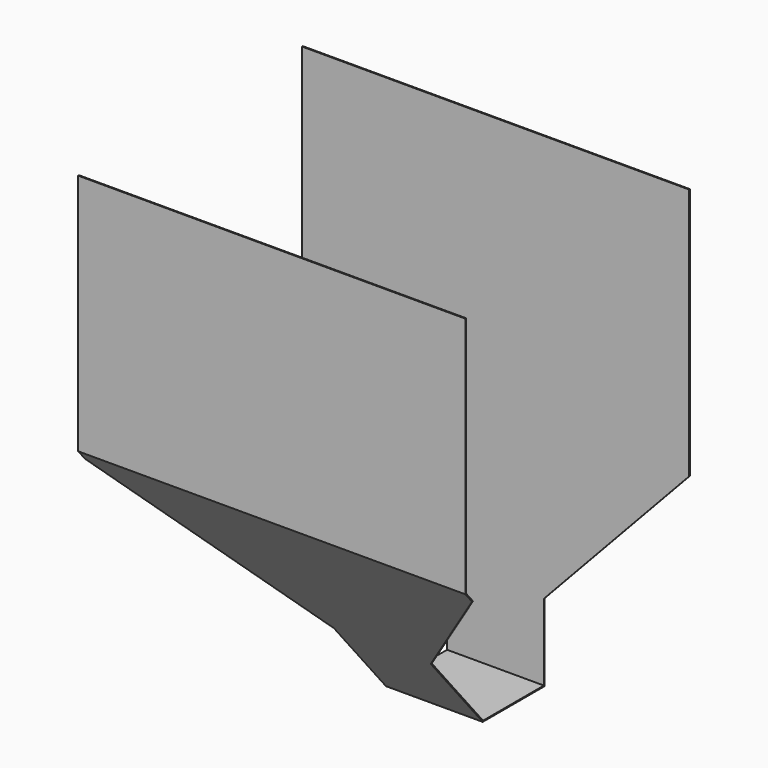
from build123d import *

# Parameters (mm, degrees)
F1_DEPTH = 400
F3_DEPTH = 290.001


# Not quite as in the source:
# - a feature names something its author has since deleted; it is built from what else it names


with BuildPart() as f1:
    # F0 (on Right) → F1 (new body)
    with BuildSketch(Plane.YZ):
        Polygon((-80, 0), (0, 0), (0, 501), (-1, 501), (-1, 1), (-79.5336923418, 1), (-289, 250.6322246791), (-289, 501), (-290, 501), (-290, 250.2682544448), align=None)
    extrude(amount=-F1_DEPTH)

    # F2 (on face) → F3 (cut, through all)
    with BuildSketch(Plane(origin=(0, 0, 0), x_dir=(-1, 0, 0), z_dir=(0, 1, 0))):
        Polygon((400, 0), (400, 240), (250, 80), (250, 0), align=None)
        Polygon((0, 0), (150, 0), (150, 80), (0, 240), align=None)
    extrude(amount=-F3_DEPTH, mode=Mode.SUBTRACT)


solid = f1.part
